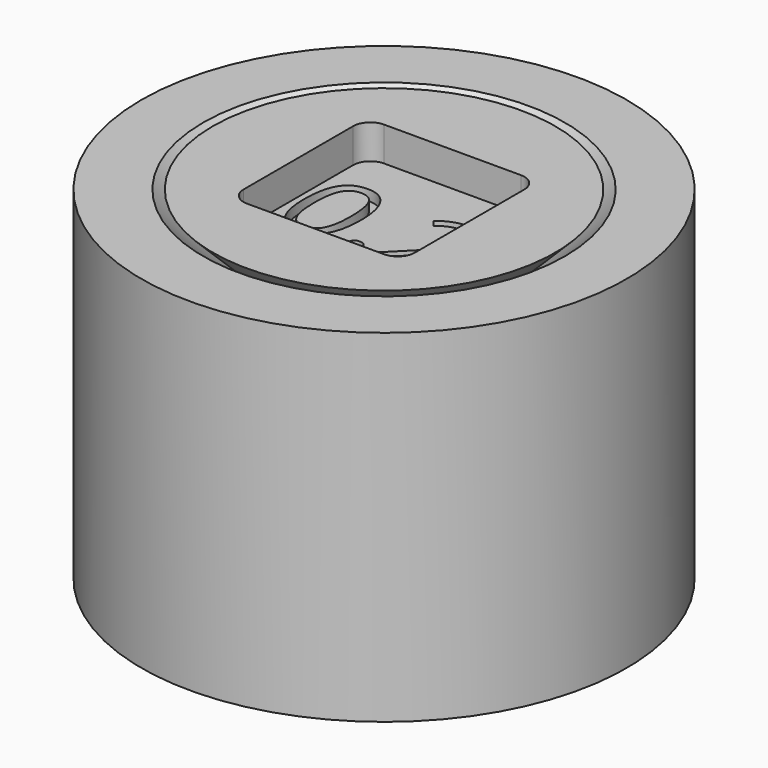
from build123d import *

# Parameters (mm, degrees)
F4_DEPTH     = 1
F5_TEXT_SIZE = 3.5191905862
F6_DEPTH     = 1.3


# Not quite as in the source:
# - Text() gives the source's letters only with a copy of the font that has no kerning and outlines rounded to 1/6400 em; it was checked with that copy


with BuildPart() as f1:
    # F0 (on Front) → F1 (revolve)
    with BuildSketch(Plane.XZ):
        with BuildLine():
            Line((-5, 0), (0, 0))
            Line((0, 0), (0, 10))
            Line((0, 10), (-5, 10))
            Line((-5, 10), (-2.7928932188, 7.7928932188))
            ThreePointArc((-2.7928932188, 7.7928932188), (-2.5761204675, 7.46846987), (-2.5, 7.0857864376))
            Line((-2.5, 7.0857864376), (-2.5, 2.9142135624))
            ThreePointArc((-2.5, 2.9142135624), (-2.5761204675, 2.53153013), (-2.7928932188, 2.2071067812))
            Line((-2.7928932188, 2.2071067812), (-5, 0))
        make_face()
    revolve(axis=Axis((0, 0, 5), (0, 0, 1)))

    # F3 (on face) → F4 (cut)
    with BuildSketch(Plane.XY.offset(10)):
        with BuildLine():
            Line((2, 2.5), (-2, 2.5))
            ThreePointArc((-2, 2.5), (-2.3535533906, 2.3535533906), (-2.5, 2))
            Line((-2.5, 2), (-2.5, -2))
            ThreePointArc((-2.5, -2), (-2.3535533906, -2.3535533906), (-2, -2.5))
            Line((-2, -2.5), (2, -2.5))
            ThreePointArc((2, -2.5), (2.3535533906, -2.3535533906), (2.5, -2))
            Line((2.5, -2), (2.5, 2))
            ThreePointArc((2.5, 2), (2.3535533906, 2.3535533906), (2, 2.5))
        make_face()
    extrude(amount=-F4_DEPTH, mode=Mode.SUBTRACT)

    # F5 (on offset) → F6 (cut)
    with BuildSketch(Plane.XY.offset(10)):
        with Locations((-2.5, -1.266908611)):
            Text('0.2', F5_TEXT_SIZE, font='Open Sans', text_align=(TextAlign.LEFT, TextAlign.BOTTOM))
    extrude(amount=-F6_DEPTH, mode=Mode.SUBTRACT)


with BuildPart() as f1b:
    # F0 (on Front) → F1, piece 2 (revolve)
    with BuildSketch(Plane.XZ):
        with BuildLine():
            Line((-7.0828427125, 10), (-7.0828427125, 0))
            Line((-7.0828427125, 0), (-5.2828427125, 0))
            Line((-5.2828427125, 0), (-2.9928932188, 2.2899494937))
            ThreePointArc((-2.9928932188, 2.2899494937), (-2.7761204675, 2.6143728425), (-2.7, 2.9970562748))
            Line((-2.7, 2.9970562748), (-2.7, 7.0029437252))
            ThreePointArc((-2.7, 7.0029437252), (-2.7761204675, 7.3856271575), (-2.9928932188, 7.7100505063))
            Line((-2.9928932188, 7.7100505063), (-5.2828427125, 10))
            Line((-5.2828427125, 10), (-7.0828427125, 10))
        make_face()
    revolve(axis=Axis((0, 0, 5), (0, 0, 1)))


solid = Compound([f1.part, f1b.part])
